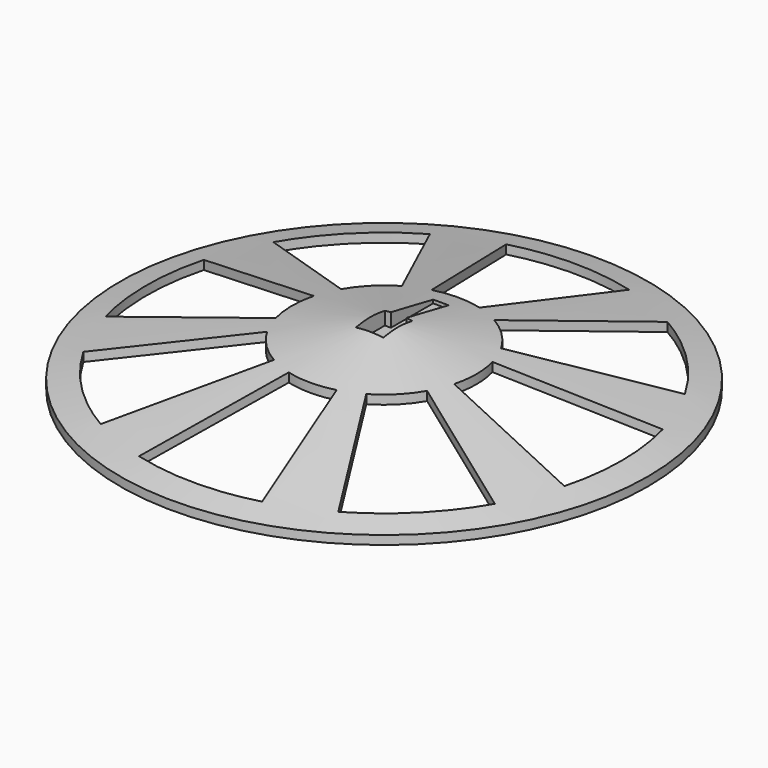
from build123d import *

# Parameters (mm, degrees)
F3_W         = 3.5
F3_H         = 12
F4_DEPTH     = 4
F5_T         = 2
F5_T3_DEPTH  = 6.9649879228
F5_T5_DEPTH  = 12.25
F5_T7_DEPTH  = 10.25
F5_T9_DEPTH  = 5.375
F5_T11_DEPTH = 16
F5_T13_DEPTH = 4.7560633483
F5_T15_DEPTH = 7.5
F5_T17_DEPTH = 5.375
F7_DEPTH     = 25


# Not quite as in the source:
# - a shell that OpenCascade refuses in one call is made with other operations: the cavity is built on its own and cut out


with BuildPart() as f1:
    # F0 (on Front) → F1 (revolve)
    with BuildSketch(Plane.XZ):
        Polygon((60, 2), (0, 14), (0, 0), (60, 0), align=None)
    revolve(axis=Axis((0, 0, 7), (0, 0, -1)))

    # F3 (on offset) → F4 (cut)
    with BuildSketch(Plane.XY.offset(14)):
        Polygon((3.125, -4.125), (3.125, 4.125), (1.75, 4.125), (-1.75, 4.125), (-3.125, 4.125), (-3.125, -4.125), align=None)
        with Locations((0, 10.125)):
            Rectangle(F3_W, F3_H)
    extrude(amount=-F4_DEPTH, mode=Mode.SUBTRACT)

    # F5: shell of thickness 2, made by hand


with BuildPart() as f5_core1:
    # F5_t2: copy of F1
    add(f1.part)

    # the walls: a layer under each face that stays
    f5_faces = [f5_core1.faces().sort_by_distance(p)[0] for p in [
        (-31.5412459886, 0, 7.6917508023),
        (3.125, 0, 11.6875),
        (0, -4.125, 11.5875),
        (-3.125, 0, 11.6875),
        (-2.4375, 4.125, 11.5519137918),
        (-1.75, 10.125, 11.5519137918),
        (0, 16.125, 10.3875),
        (1.75, 10.125, 11.5519137918),
        (2.4375, 4.125, 11.5519137918),
        (-60, 0, 1),
        (0, 6, 10),
    ]]
    thicken(f5_faces, amount=-F5_T, mode=Mode.SUBTRACT)

    # F5_s4 → F5_t3 (cut)
    with BuildSketch(Plane.XY.offset(8)):
        Polygon((3.105, 4.105), (5.125, 4.125), (5.125, 6.125), (3.125, 6.125), align=None)
        Polygon((3.105, -4.105), (5.125, -4.125), (5.125, -6.125), (3.125, -6.125), align=None)
        Polygon((-3.105, -4.105), (-3.125, -6.125), (-5.125, -6.125), (-5.125, -4.125), align=None)
        Polygon((-3.105, 4.105), (-5.125, 4.125), (-5.125, 6.125), (-3.125, 6.125), align=None)
    extrude(amount=F5_T3_DEPTH, mode=Mode.SUBTRACT)

    # F5_s6 → F5_t5 (cut)
    with BuildSketch(Plane.XZ.offset(-6.125)):
        Polygon((3.105, 10.02), (5.125, 10), (5.125, 8), (3.125, 8), align=None)
        Polygon((-3.105, 10.02), (-5.125, 10), (-5.125, 8), (-3.125, 8), align=None)
    extrude(amount=F5_T5_DEPTH, mode=Mode.SUBTRACT)

    # F5_s8 → F5_t7 (cut)
    with BuildSketch(Plane.YZ.offset(-5.125)):
        Polygon((-4.105, 10.02), (-6.125, 10), (-6.125, 8), (-4.125, 8), align=None)
    extrude(amount=F5_T7_DEPTH, mode=Mode.SUBTRACT)

    # F5_s10 → F5_t9 (cut)
    with BuildSketch(Plane.YZ.offset(-5.125)):
        Polygon((4.105, 10.02), (6.125, 10), (6.125, 8), (4.125, 8), align=None)
    extrude(amount=F5_T9_DEPTH, mode=Mode.SUBTRACT)

    # F5_s12 → F5_t11 (cut)
    with BuildSketch(Plane.XZ.offset(-18.125)):
        Polygon((-1.73, 10.02), (-3.75, 10), (-3.75, 8), (-1.75, 8), align=None)
        Polygon((1.73, 10.02), (3.75, 10), (3.75, 8), (1.75, 8), align=None)
    extrude(amount=F5_T11_DEPTH, mode=Mode.SUBTRACT)

    # F5_s14 → F5_t13 (cut)
    with BuildSketch(Plane.XY.offset(8)):
        Polygon((-1.73, 16.105), (-3.75, 16.125), (-3.75, 18.125), (-1.75, 18.125), align=None)
        Polygon((1.73, 16.105), (1.75, 18.125), (3.75, 18.125), (3.75, 16.125), align=None)
    extrude(amount=F5_T13_DEPTH, mode=Mode.SUBTRACT)

    # F5_s16 → F5_t15 (cut)
    with BuildSketch(Plane.YZ.offset(-3.75)):
        Polygon((16.105, 10.02), (18.125, 10), (18.125, 8), (16.125, 8), align=None)
    extrude(amount=F5_T15_DEPTH, mode=Mode.SUBTRACT)

    # F5_s18 → F5_t17 (cut)
    with BuildSketch(Plane.YZ.offset(-0.25)):
        Polygon((4.105, 10.02), (6.125, 10), (6.125, 8), (4.125, 8), align=None)
    extrude(amount=F5_T17_DEPTH, mode=Mode.SUBTRACT)


with BuildPart() as f1_1:
    add(f1.part)

    # what is left inside the walls is the cavity
    f5_cavity = [f5_core1.part.solids().sort_by_distance(p)[0] for p in [
        (0, 19.333333, 0.02),
    ]]
    add(f5_cavity, mode=Mode.SUBTRACT)

    # F6 (on offset) → F7 (cut)
    with BuildSketch(Plane.XY.offset(14)):
        with BuildLine():
            ThreePointArc((5.4351999472, -20.2844423521), (0, -21), (-5.4351999472, -20.2844423521))
            Line((-5.4351999472, -20.2844423521), (-13.9762284355, -52.1599946196))
            ThreePointArc((-13.9762284355, -52.1599946196), (0, -54), (13.9762284355, -52.1599946196))
            Line((13.9762284355, -52.1599946196), (5.4351999472, -20.2844423521))
        make_face()
        with BuildLine():
            ThreePointArc((18.1865334795, -10.5), (14.8492424049, -14.8492424049), (10.5, -18.1865334795))
            Line((10.5, -18.1865334795), (27, -46.7653718044))
            ThreePointArc((27, -46.7653718044), (38.1837661841, -38.1837661841), (46.7653718044, -27))
            Line((46.7653718044, -27), (18.1865334795, -10.5))
        make_face()
        with BuildLine():
            ThreePointArc((20.2844423521, 5.4351999472), (21, 0), (20.2844423521, -5.4351999472))
            Line((20.2844423521, -5.4351999472), (52.1599946196, -13.9762284355))
            ThreePointArc((52.1599946196, -13.9762284355), (54, 0), (52.1599946196, 13.9762284355))
            Line((52.1599946196, 13.9762284355), (20.2844423521, 5.4351999472))
        make_face()
        with BuildLine():
            ThreePointArc((10.5, 18.1865334795), (14.8492424049, 14.8492424049), (18.1865334795, 10.5))
            Line((18.1865334795, 10.5), (46.7653718044, 27))
            ThreePointArc((46.7653718044, 27), (38.1837661841, 38.1837661841), (27, 46.7653718044))
            Line((27, 46.7653718044), (10.5, 18.1865334795))
        make_face()
        with BuildLine():
            ThreePointArc((-5.4351999472, 20.2844423521), (0, 21), (5.4351999472, 20.2844423521))
            Line((5.4351999472, 20.2844423521), (13.9762284355, 52.1599946196))
            ThreePointArc((13.9762284355, 52.1599946196), (0, 54), (-13.9762284355, 52.1599946196))
            Line((-13.9762284355, 52.1599946196), (-5.4351999472, 20.2844423521))
        make_face()
        with BuildLine():
            ThreePointArc((-18.1865334795, 10.5), (-14.8492424049, 14.8492424049), (-10.5, 18.1865334795))
            Line((-10.5, 18.1865334795), (-27, 46.7653718044))
            ThreePointArc((-27, 46.7653718044), (-38.1837661841, 38.1837661841), (-46.7653718044, 27))
            Line((-46.7653718044, 27), (-18.1865334795, 10.5))
        make_face()
        with BuildLine():
            ThreePointArc((-20.2844423521, -5.4351999472), (-21, 0), (-20.2844423521, 5.4351999472))
            Line((-20.2844423521, 5.4351999472), (-52.1599946196, 13.9762284355))
            ThreePointArc((-52.1599946196, 13.9762284355), (-54, 0), (-52.1599946196, -13.9762284355))
            Line((-52.1599946196, -13.9762284355), (-20.2844423521, -5.4351999472))
        make_face()
        with BuildLine():
            ThreePointArc((-10.5, -18.1865334795), (-14.8492424049, -14.8492424049), (-18.1865334795, -10.5))
            Line((-18.1865334795, -10.5), (-46.7653718044, -27))
            ThreePointArc((-46.7653718044, -27), (-38.1837661841, -38.1837661841), (-27, -46.7653718044))
            Line((-27, -46.7653718044), (-10.5, -18.1865334795))
        make_face()
    extrude(amount=-F7_DEPTH, mode=Mode.SUBTRACT)


solid = f1_1.part
